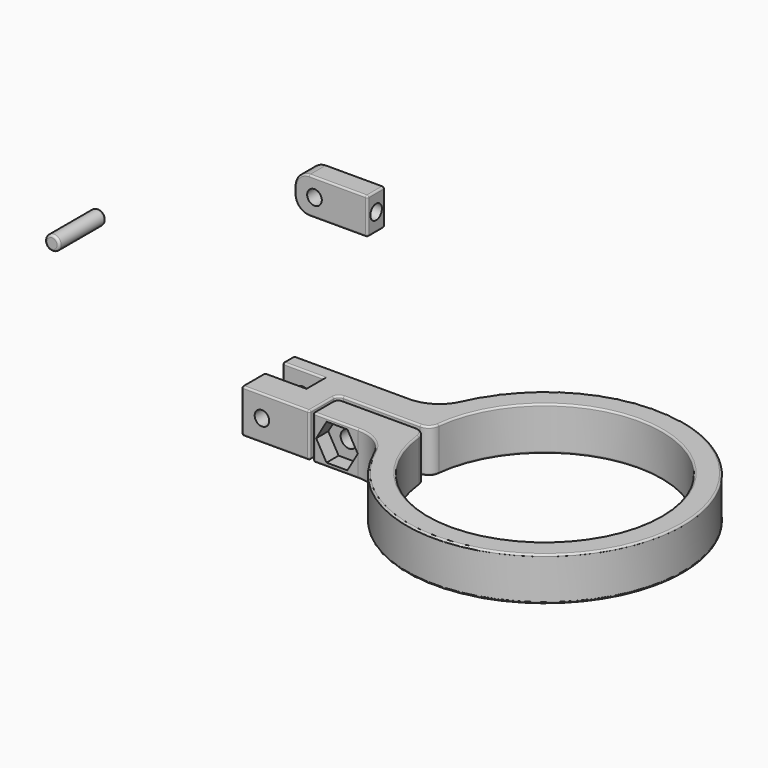
from build123d import *

# Parameters (mm, degrees)
F1_DEPTH      = 9.525
F4_DEPTH      = 4.8768
F2_R          = 1.5875
F5_DEPTH      = 16.2052
F5_DEPTH_BACK = 25.4
F8_R          = 0.381
F2_R_2        = 1.6002
F9_DEPTH      = 4.7498
F10_R         = 0.381
F11_R         = 1.5875
F12_DEPTH     = 7.112
F13_R         = 1.5875
F14_DEPTH     = 12.7
F15_R         = 0.508
F6_R          = 1.8415
F16_DEPTH     = 25.4
F6_R_2        = 3.302
F17_DEPTH     = 2.54
F18_DEPTH     = 3.302
F19_R         = 3.3528
F19_R_2       = 1.5875
F20_DEPTH     = 1.4732


# Not quite as in the source:
# - ends of sketch curves that miss each other by under 0.0002 mm in the source are joined
# - a feature names something its author has since deleted; it is built from what else it names


with BuildPart() as f1:
    # F0 (on Top) → F1 (new body)
    with BuildSketch(Plane.XY):
        with BuildLine():
            ThreePointArc((-28.3979874, 20.30984), (-28.2817454038, 20.0292069962), (-28.0011124, 19.912965))
            Line((-28.0011124, 19.912965), (-19.370929, 19.912965))
            Line((-19.370929, 19.912965), (-19.370929, 15.099665))
            Line((-19.370929, 15.099665), (-28.0011124, 15.099665))
            ThreePointArc((-28.0011124, 15.099665), (-28.2817454038, 14.9834230038), (-28.3979874, 14.70279))
            Line((-28.3979874, 14.70279), (-28.3979874, 9.14654))
            ThreePointArc((-28.3979874, 9.14654), (-28.2817454038, 8.8659069962), (-28.0011124, 8.749665))
            Line((-28.0011124, 8.749665), (-14.0088874, 8.749665))
            ThreePointArc((-14.0088874, 8.749665), (-13.7282543962, 8.8659069962), (-13.6120124, 9.14654))
            Line((-13.6120124, 9.14654), (-13.6120124, 15.3234898))
            ThreePointArc((-13.6120124, 15.3234898), (-13.2632864114, 16.1653888113), (-12.4213874, 16.5141148))
            Line((-12.4213874, 16.5141148), (4.339463, 16.5141148))
            ThreePointArc((4.339463, 16.5141148), (5.9336039467, 17.1264481246), (6.7078850502, 18.648527699))
            ThreePointArc((6.7078850502, 18.648527699), (57.4215819635, 16.0994244683), (6.7264293291, 13.2052061477))
            ThreePointArc((6.7264293291, 13.2052061477), (5.9478389323, 14.7165758926), (4.3597322, 15.3234898))
            Line((4.3597322, 15.3234898), (-11.6276374, 15.3234898))
            ThreePointArc((-11.6276374, 15.3234898), (-12.4695364114, 14.9747638113), (-12.8182624, 14.1328648))
            Line((-12.8182624, 14.1328648), (-12.8182624, 9.14654))
            ThreePointArc((-12.8182624, 9.14654), (-12.7020204038, 8.8659069962), (-12.4213874, 8.749665))
            Line((-12.4213874, 8.749665), (-2.9677106, 8.749665))
            ThreePointArc((-2.9677106, 8.749665), (1.384528339, 7.4500805213), (4.3116076755, 3.9768816847))
            ThreePointArc((4.3116076755, 3.9768816847), (62.1841201628, 16.0940335016), (4.2473111459, 27.8999190802))
            ThreePointArc((4.2473111459, 27.8999190802), (1.3211481307, 24.399270034), (-3.0489144, 23.087965))
            Line((-3.0489144, 23.087965), (-28.0011124, 23.087965))
            ThreePointArc((-28.0011124, 23.087965), (-28.2817454038, 22.9717230038), (-28.3979874, 22.69109))
            Line((-28.3979874, 22.69109), (-28.3979874, 20.30984))
        make_face()
    extrude(amount=F1_DEPTH)

    # F3 (on face) → F4 (join)
    with BuildSketch(Plane(origin=(0, 15.099665, 0), x_dir=(-1, 0, 0), z_dir=(0, 1, 0))):
        with BuildLine():
            ThreePointArc((21.3352564153, 0.67564), (19.9027023134, 1.9575586715), (19.370929, 3.80492))
            Line((19.370929, 3.80492), (19.370929, 0))
            Line((19.370929, 0), (22.0108964153, 0))
            ThreePointArc((22.0108964153, 0), (21.8130060409, 0.4777496256), (21.3352564153, 0.67564))
        make_face()
    extrude(amount=F4_DEPTH)

    # F2 (on face) → F5 (cut, two sides)
    with BuildSketch(Plane(origin=(0, 23.087965, 0), x_dir=(-1, 0, 0), z_dir=(0, 1, 0))) as f5_sk:
        with Locations((23.9809274, 4.7625)):
            Circle(F2_R)
    extrude(amount=-F5_DEPTH, mode=Mode.SUBTRACT)
    extrude(f5_sk.sketch, amount=F5_DEPTH_BACK, mode=Mode.SUBTRACT)

    # F8
    f8_edges = [f1.edges().sort_by_distance(p)[0] for p in [
        (1.384528, 7.450081, 0),
        (1.384528, 7.450081, 9.525),
        (-19.370929, 17.506315, 9.525),
    ]]
    fillet(f8_edges, radius=F8_R)

    # F6 (on face) → F16 (cut)
    with BuildSketch(Plane(origin=(0, 23.087965, 0), x_dir=(-1, 0, 0), z_dir=(0, 1, 0))):
        with Locations((7.5979274, 4.7498)):
            Circle(F6_R)
    extrude(amount=-F16_DEPTH, mode=Mode.SUBTRACT)

    # F6 (on face) → F17 (cut)
    with BuildSketch(Plane(origin=(0, 23.087965, 0), x_dir=(-1, 0, 0), z_dir=(0, 1, 0))):
        with Locations((7.5979274, 4.7498)):
            Circle(F6_R_2)
        with Locations((7.5979274, 4.7498)):
            Circle(F6_R, mode=Mode.SUBTRACT)
    extrude(amount=-F17_DEPTH, mode=Mode.SUBTRACT)

    # F7 (on face) → F18 (cut)
    with BuildSketch(Plane.XZ.offset(-8.749665)):
        Polygon((-9.8811078409, 0.8186789884), (-5.3350669591, 0.806947231), (-3.0518865182, 4.7380682425), (-5.3147469591, 8.6809210116), (-9.8607878409, 8.692652769), (-12.1439682818, 4.7615317575), align=None)
    extrude(amount=-F18_DEPTH, mode=Mode.SUBTRACT)

    # F19 (on face) → F20 (cut)
    with BuildSketch(Plane(origin=(0, 15.099665, 0), x_dir=(-1, 0, 0), z_dir=(0, 1, 0))):
        with Locations((23.9809274, 4.7625)):
            Circle(F19_R)
        with Locations((23.9809274, 4.7625)):
            Circle(F19_R_2, mode=Mode.SUBTRACT)
    extrude(amount=-F20_DEPTH, mode=Mode.SUBTRACT)


with BuildPart() as f9:
    # F2 (on face) → F9 (new body)
    with BuildSketch(Plane(origin=(0, 23.087965, 0), x_dir=(-1, 0, 0), z_dir=(0, 1, 0))):
        with BuildLine():
            Line((25.1239274, 45.3445153343), (12.8303274, 45.3445153343))
            ThreePointArc((12.8303274, 45.3445153343), (12.5429592041, 45.2254835301), (12.4239274, 44.9381153343))
            Line((12.4239274, 44.9381153343), (12.4239274, 37.8261153343))
            ThreePointArc((12.4239274, 37.8261153343), (12.5429592041, 37.5387471384), (12.8303274, 37.4197153343))
            Line((12.8303274, 37.4197153343), (25.1239274, 37.4197153343))
            ThreePointArc((25.1239274, 37.4197153343), (27.3689914303, 38.349651304), (28.2989274, 40.5947153343))
            Line((28.2989274, 40.5947153343), (28.2989274, 42.1695153343))
            ThreePointArc((28.2989274, 42.1695153343), (27.3689914303, 44.4145793645), (25.1239274, 45.3445153343))
        make_face()
        with Locations((23.9809274, 41.3821153343)):
            Circle(F2_R_2, mode=Mode.SUBTRACT)
    extrude(amount=F9_DEPTH)

    # F10
    f10_edges = [f9.edges().sort_by_distance(p)[0] for p in [
        (-18.977127, 27.837765, 37.419715),
        (-18.977127, 23.087965, 37.419715),
        (-12.423927, 25.462865, 44.938115),
        (-12.423927, 25.462865, 37.826115),
        (-12.423927, 23.087965, 41.382115),
        (-12.423927, 27.837765, 41.382115),
    ]]
    fillet(f10_edges, radius=F10_R)

    # F11 (on face) → F12 (cut)
    with BuildSketch(Plane.YZ.offset(-12.4239274)):
        with Locations((25.462865, 41.3821153343)):
            Circle(F11_R)
    extrude(amount=-F12_DEPTH, mode=Mode.SUBTRACT)


with BuildPart() as f14:
    # F13 (on Front) → F14 (new body)
    with BuildSketch(Plane.XZ):
        with Locations((-52.6410378516, 37.7627648413)):
            Circle(F13_R)
    extrude(amount=F14_DEPTH)

    # F15
    f15_edges = [f14.edges().sort_by_distance(p)[0] for p in [
        (-54.228538, 0, 37.762765),
        (-54.228538, -12.7, 37.762765),
    ]]
    fillet(f15_edges, radius=F15_R)


solid = Compound([f1.part, f9.part, f14.part])
